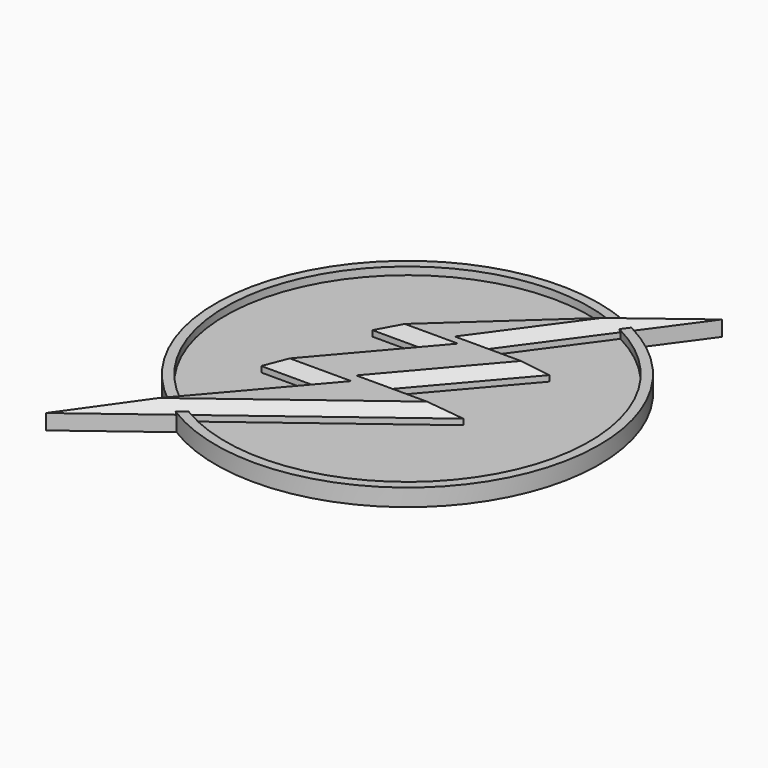
from build123d import *

# Parameters (mm, degrees)
F0_R          = 47.5
F1_DEPTH      = 2.5
F0_R_2        = 50
F2_DEPTH      = 4.5
F4_DEPTH      = 2.5
F5_DEPTH      = 2.5
F6_DEPTH      = 2.5
F7_DEPTH      = 2.5
F8_DEPTH      = 2.5
F9_DEPTH      = 1.5
F10_T4_DEPTH  = 97.8665217368
F10_S5_R      = 47.5
F10_T6_DEPTH  = 52
F10_T11_DEPTH = 97.8665217368
F10_S12_R     = 47.5
F10_T13_DEPTH = 52
F10_T18_DEPTH = 97.8665217368
F10_S19_R     = 47.5
F10_T20_DEPTH = 52
F10_S22_R     = 50
F10_T23_DEPTH = 52
F10_T27_DEPTH = 97.8665217368
F10_S29_R     = 50
F10_T30_DEPTH = 52
F10_T34_DEPTH = 97.8665217368
F10_S36_R     = 50
F10_T37_DEPTH = 52
F11_T4_DEPTH  = 71.4627253186
F11_S6_R      = 50
F11_T7_DEPTH  = 38
F11_T11_DEPTH = 71.4627253186
F11_S13_R     = 50
F11_T14_DEPTH = 38
F11_T18_DEPTH = 71.4627253186
F11_S19_R     = 47.5
F11_T20_DEPTH = 38
F11_S22_R     = 50
F11_T23_DEPTH = 38
F11_T27_DEPTH = 71.4627253186
F11_S29_R     = 47.5
F11_T30_DEPTH = 38
F11_T35_DEPTH = 71.4627253186
F11_S37_R     = 47.5
F11_T38_DEPTH = 38
F12_SIZE      = 2.5
F13_T4_DEPTH  = 32.1736802215
F13_T9_DEPTH  = 32.1736802215
F14_SIZE      = 2.5
F15_SIZE      = 2.5
F16_T1_DEPTH  = 21.3180204906
F16_T6_DEPTH  = 9.7203833333
F17_SIZE      = 2.5
F18_T4_DEPTH  = 80.4724206
F18_S5_R      = 47.5
F18_T6_DEPTH  = 43
F18_T11_DEPTH = 80.4724206
F18_S12_R     = 47.5
F18_T13_DEPTH = 43
F18_T18_DEPTH = 80.4724206
F18_S19_R     = 50
F18_T20_DEPTH = 43
F18_S21_R     = 47.5
F18_T22_DEPTH = 43
F18_T27_DEPTH = 80.4724206
F18_S28_R     = 50
F18_T29_DEPTH = 43
F18_T34_DEPTH = 80.4724206
F18_S35_R     = 50
F18_T36_DEPTH = 43
F19_T4_DEPTH  = 67.1181390524
F19_S5_R      = 47.5
F19_T6_DEPTH  = 36
F19_T11_DEPTH = 67.1181390524
F19_T17_DEPTH = 67.1181390524
F19_S18_R     = 50
F19_T19_DEPTH = 36


# Not quite as in the source:
# - a fillet or chamfer that OpenCascade refuses, or shapes differently, is made with other operations: its cross-section is extruded or revolved along the edge and cut away or added


with BuildPart() as f1:
    # F0 (on Top) → F1 (new body)
    with BuildSketch(Plane.XY):
        Circle(F0_R)
    extrude(amount=F1_DEPTH)

    # F0 (on Top) → F2 (join)
    with BuildSketch(Plane.XY):
        Circle(F0_R_2)
        Circle(F0_R, mode=Mode.SUBTRACT)
    extrude(amount=F2_DEPTH)

    # F3 (on face) → F4 (join)
    with BuildSketch(Plane.XY.offset(2.5)):
        with BuildLine():
            ThreePointArc((21.7132493209, 42.2467135281), (19.6123250887, 43.2620700454), (17.4640719677, 44.173025596))
            Line((17.4640719677, 44.173025596), (-18.3086600155, 11.4598022774))
            Line((-18.3086600155, 11.4598022774), (-3.4198469948, 11.4598022774))
            Line((-3.4198469948, 11.4598022774), (-26.0993205011, -15.0284366682))
            Line((-26.0993205011, -15.0284366682), (-10.0752310827, -15.0284366682))
            Line((-10.0752310827, -15.0284366682), (-29.2512131204, -37.4248117027))
            ThreePointArc((-29.2512131204, -37.4248117027), (-26.6854575008, -39.29550048), (-24.0004517017, -40.990588165))
            Line((-24.0004517017, -40.990588165), (20.5448437482, -7.452824153))
            Line((20.5448437482, -7.452824153), (0, -7.452824153))
            Line((0, -7.452824153), (22.2159207014, 18.4940134476))
            Line((22.2159207014, 18.4940134476), (4.4441488571, 18.4940134476))
            Line((4.4441488571, 18.4940134476), (21.7132493209, 42.2467135281))
        make_face()
    extrude(amount=F4_DEPTH)

    # F3 (on face) → F5 (join)
    with BuildSketch(Plane.XY.offset(2.5)):
        with BuildLine():
            ThreePointArc((-24.0004517017, -40.990588165), (-26.6854575008, -39.29550048), (-29.2512131204, -37.4248117027))
            Line((-29.2512131204, -37.4248117027), (-47.3672765296, -58.5832665585))
            Line((-47.3672765296, -58.5832665585), (-24.0004517017, -40.990588165))
        make_face()
    extrude(amount=F5_DEPTH)

    # F3 (on face) → F6 (join)
    with BuildSketch(Plane.XY.offset(2.5)):
        with BuildLine():
            Line((21.7132493209, 42.2467135281), (34.321565181, 59.5887601376))
            Line((34.321565181, 59.5887601376), (17.4640719677, 44.173025596))
            ThreePointArc((17.4640719677, 44.173025596), (19.6123250887, 43.2620700454), (21.7132493209, 42.2467135281))
        make_face()
    extrude(amount=F6_DEPTH)

    # F3 (on face) → F7 (join)
    with BuildSketch(Plane.XY.offset(2.5)):
        with BuildLine():
            ThreePointArc((-24.0004517017, -40.990588165), (-26.6854575008, -39.29550048), (-29.2512131204, -37.4248117027))
            Line((-29.2512131204, -37.4248117027), (-47.3672765296, -58.5832665585))
            Line((-47.3672765296, -58.5832665585), (-24.0004517017, -40.990588165))
        make_face()
    extrude(amount=-F7_DEPTH)

    # F3 (on face) → F8 (join)
    with BuildSketch(Plane.XY.offset(2.5)):
        with BuildLine():
            Line((21.7132493209, 42.2467135281), (34.321565181, 59.5887601376))
            Line((34.321565181, 59.5887601376), (17.4640719677, 44.173025596))
            ThreePointArc((17.4640719677, 44.173025596), (19.6123250887, 43.2620700454), (21.7132493209, 42.2467135281))
        make_face()
    extrude(amount=-F8_DEPTH)

    # F9 (add): a face of the model
    f9_faces = [f1.faces().sort_by_distance(p)[0] for p in [
        (-3.1603414311, -1.3488112802, 5),
    ]]
    extrude(f9_faces, amount=F9_DEPTH)

    # F10: chamfer of 2.5 on 1 edges, made by hand


with BuildPart() as f10_tool2:
    # F10_s3 → F10_t4 (new body)
    with BuildSketch(Plane(origin=(14.6672771585, 11.0428649103, 0), x_dir=(0, 0, 1), z_dir=(-0.7988899275, -0.6014772512, 0))):
        Polygon((6.5, -15.8112422913), (4, -18.3112422913), (6.5, -18.3112422913), align=None)
    extrude(amount=F10_T4_DEPTH)

    # F10_s5 → F10_t6 (intersect, symmetric)
    with BuildSketch(Plane.XY.offset(5.2)):
        Circle(F10_S5_R)
    extrude(amount=F10_T6_DEPTH, both=True, mode=Mode.INTERSECT)

    split(bisect_by=Plane.XY.offset(4.5), keep=Keep.TOP)


with BuildPart() as f1_1:
    add(f1.part)

    # F10_t1: cut F10_tool2
    add(f10_tool2.part, mode=Mode.SUBTRACT)


with BuildPart() as f10_tool9:
    # F10_s10 → F10_t11 (new body)
    with BuildSketch(Plane(origin=(14.6672771585, 11.0428649103, 0), x_dir=(0, 0, 1), z_dir=(-0.7988899275, -0.6014772512, 0))):
        Polygon((6.5, -15.8112422913), (4, -18.3112422913), (6.5, -18.3112422913), align=None)
    extrude(amount=F10_T11_DEPTH)

    # F10_s12 → F10_t13 (intersect, symmetric)
    with BuildSketch(Plane.XY.offset(5.2)):
        Circle(F10_S12_R)
    extrude(amount=F10_T13_DEPTH, both=True, mode=Mode.INTERSECT)

    split(bisect_by=Plane.XY.offset(4.5), keep=Keep.BOTTOM)


with BuildPart() as f1_2:
    add(f1_1.part)

    # F10_t8: cut F10_tool9
    add(f10_tool9.part, mode=Mode.SUBTRACT)


with BuildPart() as f10_tool16:
    # F10_s17 → F10_t18 (new body)
    with BuildSketch(Plane(origin=(14.6672771585, 11.0428649103, 0), x_dir=(0, 0, 1), z_dir=(-0.7988899275, -0.6014772512, 0))):
        Polygon((6.5, -15.8112422913), (4, -18.3112422913), (6.5, -18.3112422913), align=None)
    extrude(amount=F10_T18_DEPTH)

    # F10_s19 → F10_t20 (cut, symmetric)
    with BuildSketch(Plane.XY.offset(5.2)):
        Circle(F10_S19_R)
    extrude(amount=F10_T20_DEPTH, both=True, mode=Mode.SUBTRACT)

    split(bisect_by=Plane.XY.offset(4.5), keep=Keep.TOP)

    # F10_s22 → F10_t23 (intersect, symmetric)
    with BuildSketch(Plane.XY.offset(5.2)):
        Circle(F10_S22_R)
    extrude(amount=F10_T23_DEPTH, both=True, mode=Mode.INTERSECT)


with BuildPart() as f1_3:
    add(f1_2.part)

    # F10_t15: cut F10_tool16
    add(f10_tool16.part, mode=Mode.SUBTRACT)


with BuildPart() as f10_tool25:
    # F10_s26 → F10_t27 (new body)
    with BuildSketch(Plane(origin=(14.6672771585, 11.0428649103, 0), x_dir=(0, 0, 1), z_dir=(-0.7988899275, -0.6014772512, 0))):
        Polygon((6.5, -15.8112422913), (4, -18.3112422913), (6.5, -18.3112422913), align=None)
    extrude(amount=F10_T27_DEPTH)

    split(bisect_by=Plane.XY.offset(4.5), keep=Keep.TOP)

    # F10_s29 → F10_t30 (cut, symmetric)
    with BuildSketch(Plane.XY.offset(5.2)):
        Circle(F10_S29_R)
    extrude(amount=F10_T30_DEPTH, both=True, mode=Mode.SUBTRACT)


with BuildPart() as f1_4:
    add(f1_3.part)

    # F10_t24: cut F10_tool25
    add(f10_tool25.part, mode=Mode.SUBTRACT)


with BuildPart() as f10_tool32:
    # F10_s33 → F10_t34 (new body)
    with BuildSketch(Plane(origin=(14.6672771585, 11.0428649103, 0), x_dir=(0, 0, 1), z_dir=(-0.7988899275, -0.6014772512, 0))):
        Polygon((6.5, -15.8112422913), (4, -18.3112422913), (6.5, -18.3112422913), align=None)
    extrude(amount=F10_T34_DEPTH)

    split(bisect_by=Plane.XY.offset(4.5), keep=Keep.BOTTOM)

    # F10_s36 → F10_t37 (cut, symmetric)
    with BuildSketch(Plane.XY.offset(5.2)):
        Circle(F10_S36_R)
    extrude(amount=F10_T37_DEPTH, both=True, mode=Mode.SUBTRACT)


with BuildPart() as f1_5:
    add(f1_4.part)

    # F10_t31: cut F10_tool32
    add(f10_tool32.part, mode=Mode.SUBTRACT)

    # F11: chamfer of 2.5 on 1 edges, made by hand


with BuildPart() as f11_tool2:
    # F11_s3 → F11_t4 (new body)
    with BuildSketch(Plane(origin=(-53.9830269669, -63.0488761968, 0), x_dir=(0, 0, 1), z_dir=(0.6503824329, 0.7596069319, 0))):
        Polygon((6.5, 4.6210158312), (4, 2.1210158312), (6.5, 2.1210158312), align=None)
    extrude(amount=F11_T4_DEPTH)

    split(bisect_by=Plane.XY.offset(4.5), keep=Keep.TOP)

    # F11_s6 → F11_t7 (cut, symmetric)
    with BuildSketch(Plane.XY.offset(5.2)):
        Circle(F11_S6_R)
    extrude(amount=F11_T7_DEPTH, both=True, mode=Mode.SUBTRACT)


with BuildPart() as f1_6:
    add(f1_5.part)

    # F11_t1: cut F11_tool2
    add(f11_tool2.part, mode=Mode.SUBTRACT)


with BuildPart() as f11_tool9:
    # F11_s10 → F11_t11 (new body)
    with BuildSketch(Plane(origin=(-53.9830269669, -63.0488761968, 0), x_dir=(0, 0, 1), z_dir=(0.6503824329, 0.7596069319, 0))):
        Polygon((6.5, 4.6210158312), (4, 2.1210158312), (6.5, 2.1210158312), align=None)
    extrude(amount=F11_T11_DEPTH)

    split(bisect_by=Plane.XY.offset(4.5), keep=Keep.BOTTOM)

    # F11_s13 → F11_t14 (cut, symmetric)
    with BuildSketch(Plane.XY.offset(5.2)):
        Circle(F11_S13_R)
    extrude(amount=F11_T14_DEPTH, both=True, mode=Mode.SUBTRACT)


with BuildPart() as f1_7:
    add(f1_6.part)

    # F11_t8: cut F11_tool9
    add(f11_tool9.part, mode=Mode.SUBTRACT)


with BuildPart() as f11_tool16:
    # F11_s17 → F11_t18 (new body)
    with BuildSketch(Plane(origin=(-53.9830269669, -63.0488761968, 0), x_dir=(0, 0, 1), z_dir=(0.6503824329, 0.7596069319, 0))):
        Polygon((6.5, 4.6210158312), (4, 2.1210158312), (6.5, 2.1210158312), align=None)
    extrude(amount=F11_T18_DEPTH)

    # F11_s19 → F11_t20 (cut, symmetric)
    with BuildSketch(Plane.XY.offset(5.2)):
        Circle(F11_S19_R)
    extrude(amount=F11_T20_DEPTH, both=True, mode=Mode.SUBTRACT)

    split(bisect_by=Plane.XY.offset(4.5), keep=Keep.TOP)

    # F11_s22 → F11_t23 (intersect, symmetric)
    with BuildSketch(Plane.XY.offset(5.2)):
        Circle(F11_S22_R)
    extrude(amount=F11_T23_DEPTH, both=True, mode=Mode.INTERSECT)


with BuildPart() as f1_8:
    add(f1_7.part)

    # F11_t15: cut F11_tool16
    add(f11_tool16.part, mode=Mode.SUBTRACT)


with BuildPart() as f11_tool25:
    # F11_s26 → F11_t27 (new body)
    with BuildSketch(Plane(origin=(-53.9830269669, -63.0488761968, 0), x_dir=(0, 0, 1), z_dir=(0.6503824329, 0.7596069319, 0))):
        Polygon((6.5, 4.6210158312), (4, 2.1210158312), (6.5, 2.1210158312), align=None)
    extrude(amount=F11_T27_DEPTH)

    split(bisect_by=Plane.XZ.offset(15.0284366682), keep=Keep.TOP)

    # F11_s29 → F11_t30 (intersect, symmetric)
    with BuildSketch(Plane.XY.offset(5.2)):
        Circle(F11_S29_R)
    extrude(amount=F11_T30_DEPTH, both=True, mode=Mode.INTERSECT)

    split(bisect_by=Plane.XY.offset(4.5), keep=Keep.TOP)


with BuildPart() as f1_9:
    add(f1_8.part)

    # F11_t24: cut F11_tool25
    add(f11_tool25.part, mode=Mode.SUBTRACT)


with BuildPart() as f11_tool33:
    # F11_s34 → F11_t35 (new body)
    with BuildSketch(Plane(origin=(-53.9830269669, -63.0488761968, 0), x_dir=(0, 0, 1), z_dir=(0.6503824329, 0.7596069319, 0))):
        Polygon((6.5, 4.6210158312), (4, 2.1210158312), (6.5, 2.1210158312), align=None)
    extrude(amount=F11_T35_DEPTH)

    split(bisect_by=Plane.XZ.offset(15.0284366682), keep=Keep.TOP)

    # F11_s37 → F11_t38 (intersect, symmetric)
    with BuildSketch(Plane.XY.offset(5.2)):
        Circle(F11_S37_R)
    extrude(amount=F11_T38_DEPTH, both=True, mode=Mode.INTERSECT)

    split(bisect_by=Plane.XY.offset(4.5), keep=Keep.BOTTOM)


with BuildPart() as f1_10:
    add(f1_9.part)

    # F11_t32: cut F11_tool33
    add(f11_tool33.part, mode=Mode.SUBTRACT)

    # F12
    f12_edges = [f1_10.edges().sort_by_distance(p)[0] for p in [
        (8.194205, -7.452824, 6.5),
    ]]
    chamfer(f12_edges, length=F12_SIZE)

    # F13: chamfer of 2.5 on 1 edges, made by hand


with BuildPart() as f13_tool2:
    # F13_s3 → F13_t4 (new body)
    with BuildSketch(Plane.YZ.offset(-32.528527971)):
        Polygon((-12.5284366682, 6.5), (-15.0284366682, 4), (-15.0284366682, 6.5), align=None)
    extrude(amount=F13_T4_DEPTH)

    split(bisect_by=Plane(origin=(1.6111383281, -1.3794714365, 0), x_dir=(0, 0, 1), z_dir=(-0.7596069319, 0.6503824329, 0)), keep=Keep.TOP)


with BuildPart() as f1_11:
    add(f1_10.part)

    # F13_t1: cut F13_tool2
    add(f13_tool2.part, mode=Mode.SUBTRACT)


with BuildPart() as f13_tool7:
    # F13_s8 → F13_t9 (new body)
    with BuildSketch(Plane.YZ.offset(-32.528527971)):
        Polygon((-12.5284366682, 6.5), (-15.0284366682, 4), (-15.0284366682, 6.5), align=None)
    extrude(amount=F13_T9_DEPTH)

    split(bisect_by=Plane(origin=(-0.7136446998, 0.6110291475, 0.9394920844), x_dir=(-0.6503824329, -0.7596069319, 0), z_dir=(-0.5371232126, 0.4598898286, 0.7071067812)), keep=Keep.TOP)

    split(bisect_by=Plane(origin=(1.6111383281, -1.3794714365, 0), x_dir=(0, 0, 1), z_dir=(0.7596069319, -0.6503824329, 0)), keep=Keep.TOP)


with BuildPart() as f1_12:
    add(f1_11.part)

    # F13_t6: cut F13_tool7
    add(f13_tool7.part, mode=Mode.SUBTRACT)

    # F14
    f14_edges = [f1_12.edges().sort_by_distance(p)[0] for p in [
        (-13.689322, -0.534317, 6.5),
    ]]
    chamfer(f14_edges, length=F14_SIZE)

    # F15
    f15_edges = [f1_12.edges().sort_by_distance(p)[0] for p in [
        (10.037699, 4.270595, 6.5),
    ]]
    chamfer(f15_edges, length=F15_SIZE)

    # F16: chamfer of 2.5 on 1 edges, made by hand

    # F16_s2 → F16_t1 (cut)
    with BuildSketch(Plane.YZ.offset(-24.7378674854)):
        Polygon((13.9598022774, 6.5), (11.4598022774, 4), (11.4598022774, 6.5), align=None)
    extrude(amount=F16_T1_DEPTH, mode=Mode.SUBTRACT)


with BuildPart() as f16_tool4:
    # F16_s5 → F16_t6 (new body)
    with BuildSketch(Plane.YZ.offset(-3.4198469948)):
        Polygon((13.9598022774, 6.5), (11.4598022774, 4), (11.4598022774, 6.5), align=None)
    extrude(amount=F16_T6_DEPTH)

    split(bisect_by=Plane(origin=(-5.3366160576, 4.5692596907, 7.0254967843), x_dir=(-0.6503824329, -0.7596069319, 0), z_dir=(-0.5371232126, 0.4598898286, 0.7071067812)), keep=Keep.TOP)


with BuildPart() as f1_13:
    add(f1_12.part)

    # F16_t3: cut F16_tool4
    add(f16_tool4.part, mode=Mode.SUBTRACT)

    # F17
    f17_edges = [f1_13.edges().sort_by_distance(p)[0] for p in [
        (11.684447, 18.494013, 6.5),
    ]]
    chamfer(f17_edges, length=F17_SIZE)

    # F18: chamfer of 2.5 on 1 edges, made by hand


with BuildPart() as f18_tool2:
    # F18_s3 → F18_t4 (new body)
    with BuildSketch(Plane(origin=(-6.2742203903, -5.7376096652, 0), x_dir=(0, 0, 1), z_dir=(0.7379597151, 0.6748447665, 0))):
        Polygon((6.5, -18.3123758167), (4, -20.8123758167), (6.5, -20.8123758167), align=None)
    extrude(amount=F18_T4_DEPTH)

    # F18_s5 → F18_t6 (intersect, symmetric)
    with BuildSketch(Plane.XY.offset(5.2)):
        Circle(F18_S5_R)
    extrude(amount=F18_T6_DEPTH, both=True, mode=Mode.INTERSECT)

    split(bisect_by=Plane.XY.offset(4.5), keep=Keep.TOP)


with BuildPart() as f1_14:
    add(f1_13.part)

    # F18_t1: cut F18_tool2
    add(f18_tool2.part, mode=Mode.SUBTRACT)


with BuildPart() as f18_tool9:
    # F18_s10 → F18_t11 (new body)
    with BuildSketch(Plane(origin=(-6.2742203903, -5.7376096652, 0), x_dir=(0, 0, 1), z_dir=(0.7379597151, 0.6748447665, 0))):
        Polygon((6.5, -18.3123758167), (4, -20.8123758167), (6.5, -20.8123758167), align=None)
    extrude(amount=F18_T11_DEPTH)

    # F18_s12 → F18_t13 (intersect, symmetric)
    with BuildSketch(Plane.XY.offset(5.2)):
        Circle(F18_S12_R)
    extrude(amount=F18_T13_DEPTH, both=True, mode=Mode.INTERSECT)

    split(bisect_by=Plane.XY.offset(4.5), keep=Keep.BOTTOM)


with BuildPart() as f1_15:
    add(f1_14.part)

    # F18_t8: cut F18_tool9
    add(f18_tool9.part, mode=Mode.SUBTRACT)


with BuildPart() as f18_tool16:
    # F18_s17 → F18_t18 (new body)
    with BuildSketch(Plane(origin=(-6.2742203903, -5.7376096652, 0), x_dir=(0, 0, 1), z_dir=(0.7379597151, 0.6748447665, 0))):
        Polygon((6.5, -18.3123758167), (4, -20.8123758167), (6.5, -20.8123758167), align=None)
    extrude(amount=F18_T18_DEPTH)

    # F18_s19 → F18_t20 (intersect, symmetric)
    with BuildSketch(Plane.XY.offset(5.2)):
        Circle(F18_S19_R)
    extrude(amount=F18_T20_DEPTH, both=True, mode=Mode.INTERSECT)

    # F18_s21 → F18_t22 (cut, symmetric)
    with BuildSketch(Plane.XY.offset(5.2)):
        Circle(F18_S21_R)
    extrude(amount=F18_T22_DEPTH, both=True, mode=Mode.SUBTRACT)

    split(bisect_by=Plane.XY.offset(4.5), keep=Keep.TOP)


with BuildPart() as f1_16:
    add(f1_15.part)

    # F18_t15: cut F18_tool16
    add(f18_tool16.part, mode=Mode.SUBTRACT)


with BuildPart() as f18_tool25:
    # F18_s26 → F18_t27 (new body)
    with BuildSketch(Plane(origin=(-6.2742203903, -5.7376096652, 0), x_dir=(0, 0, 1), z_dir=(0.7379597151, 0.6748447665, 0))):
        Polygon((6.5, -18.3123758167), (4, -20.8123758167), (6.5, -20.8123758167), align=None)
    extrude(amount=F18_T27_DEPTH)

    # F18_s28 → F18_t29 (cut, symmetric)
    with BuildSketch(Plane.XY.offset(5.2)):
        Circle(F18_S28_R)
    extrude(amount=F18_T29_DEPTH, both=True, mode=Mode.SUBTRACT)

    split(bisect_by=Plane.XY.offset(4.5), keep=Keep.TOP)


with BuildPart() as f1_17:
    add(f1_16.part)

    # F18_t24: cut F18_tool25
    add(f18_tool25.part, mode=Mode.SUBTRACT)


with BuildPart() as f18_tool32:
    # F18_s33 → F18_t34 (new body)
    with BuildSketch(Plane(origin=(-6.2742203903, -5.7376096652, 0), x_dir=(0, 0, 1), z_dir=(0.7379597151, 0.6748447665, 0))):
        Polygon((6.5, -18.3123758167), (4, -20.8123758167), (6.5, -20.8123758167), align=None)
    extrude(amount=F18_T34_DEPTH)

    # F18_s35 → F18_t36 (cut, symmetric)
    with BuildSketch(Plane.XY.offset(5.2)):
        Circle(F18_S35_R)
    extrude(amount=F18_T36_DEPTH, both=True, mode=Mode.SUBTRACT)

    split(bisect_by=Plane.XY.offset(4.5), keep=Keep.BOTTOM)


with BuildPart() as f1_18:
    add(f1_17.part)

    # F18_t31: cut F18_tool32
    add(f18_tool32.part, mode=Mode.SUBTRACT)

    # F19: chamfer of 2.5 on 1 edges, made by hand


with BuildPart() as f19_tool2:
    # F19_s3 → F19_t4 (new body)
    with BuildSketch(Plane(origin=(4.73478831, 6.5124415083, 0), x_dir=(0, 0, 1), z_dir=(0.5880471799, 0.808826628, 0))):
        Polygon((6.5, -9.7808065182), (4, -7.2808065182), (6.5, -7.2808065182), align=None)
    extrude(amount=F19_T4_DEPTH)

    # F19_s5 → F19_t6 (intersect, symmetric)
    with BuildSketch(Plane.XY.offset(5.2)):
        Circle(F19_S5_R)
    extrude(amount=F19_T6_DEPTH, both=True, mode=Mode.INTERSECT)

    split(bisect_by=Plane(origin=(0, 11.2470067238, 11.2470067238), x_dir=(1, 0, 0), z_dir=(0, 0.7071067812, 0.7071067812)), keep=Keep.TOP)


with BuildPart() as f1_19:
    add(f1_18.part)

    # F19_t1: cut F19_tool2
    add(f19_tool2.part, mode=Mode.SUBTRACT)


with BuildPart() as f19_tool9:
    # F19_s10 → F19_t11 (new body)
    with BuildSketch(Plane(origin=(4.73478831, 6.5124415083, 0), x_dir=(0, 0, 1), z_dir=(0.5880471799, 0.808826628, 0))):
        Polygon((6.5, -9.7808065182), (4, -7.2808065182), (6.5, -7.2808065182), align=None)
    extrude(amount=F19_T11_DEPTH)

    split(bisect_by=Plane.XY.offset(4.5), keep=Keep.TOP)

    split(bisect_by=Plane(origin=(0, 11.2470067238, 11.2470067238), x_dir=(1, 0, 0), z_dir=(0, 0.7071067812, 0.7071067812)), keep=Keep.TOP)


with BuildPart() as f1_20:
    add(f1_19.part)

    # F19_t8: cut F19_tool9
    add(f19_tool9.part, mode=Mode.SUBTRACT)


with BuildPart() as f19_tool15:
    # F19_s16 → F19_t17 (new body)
    with BuildSketch(Plane(origin=(4.73478831, 6.5124415083, 0), x_dir=(0, 0, 1), z_dir=(0.5880471799, 0.808826628, 0))):
        Polygon((6.5, -9.7808065182), (4, -7.2808065182), (6.5, -7.2808065182), align=None)
    extrude(amount=F19_T17_DEPTH)

    # F19_s18 → F19_t19 (cut, symmetric)
    with BuildSketch(Plane.XY.offset(5.2)):
        Circle(F19_S18_R)
    extrude(amount=F19_T19_DEPTH, both=True, mode=Mode.SUBTRACT)


with BuildPart() as f1_21:
    add(f1_20.part)

    # F19_t14: cut F19_tool15
    add(f19_tool15.part, mode=Mode.SUBTRACT)


solid = f1_21.part
